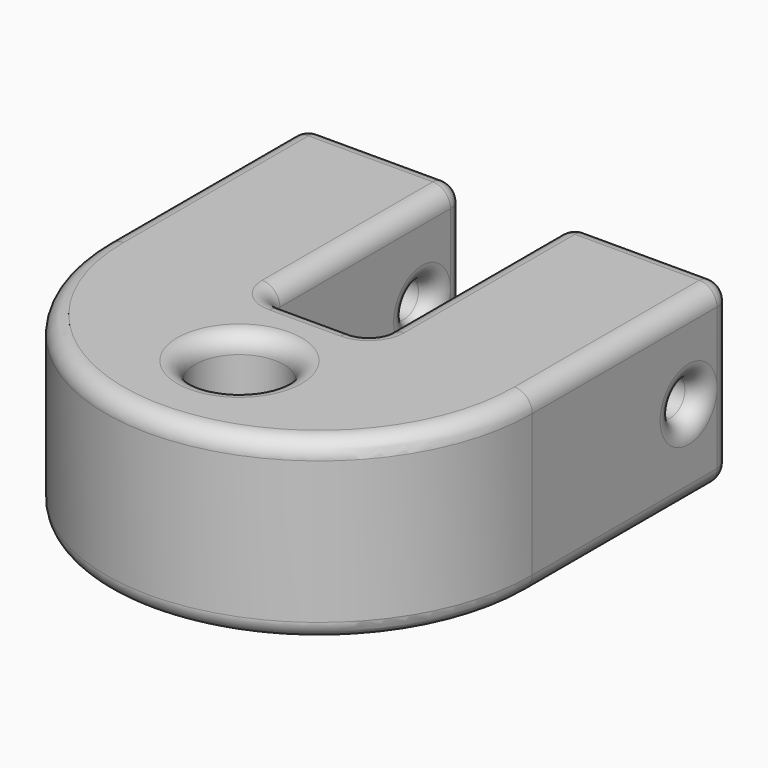
from build123d import *

# Parameters (mm, degrees)
F1_DEPTH = 50
F2_R     = 12.5
F3_DEPTH = 50.001
F4_R     = 5
F5_DEPTH = 120.001
F6_R     = 4.99999


# Not quite as in the source:
# - a fillet or chamfer is up to 0.001 mm smaller than in the source, because OpenCascade refuses the exact size


with BuildPart() as f1:
    # F0 (on Top) → F1 (new body)
    with BuildSketch(Plane.XY):
        with BuildLine():
            Line((-15, 70), (-60, 70))
            Line((-60, 70), (-60, 0))
            ThreePointArc((-60, 0), (0, -60), (60, 0))
            Line((60, 0), (60, 70))
            Line((60, 70), (15, 70))
            Line((15, 70), (15, 0))
            Line((15, 0), (-15, 0))
            Line((-15, 0), (-15, 70))
        make_face()
    extrude(amount=F1_DEPTH)

    # F2 (on face) → F3 (cut, through all)
    with BuildSketch(Plane.XY.offset(50)):
        with Locations((0, -28)):
            Circle(F2_R)
    extrude(amount=-F3_DEPTH, mode=Mode.SUBTRACT)

    # F4 (on face) → F5 (cut, through all)
    with BuildSketch(Plane.YZ.offset(60)):
        with Locations((55, 25)):
            Circle(F4_R)
    extrude(amount=-F5_DEPTH, mode=Mode.SUBTRACT)

    # F6 (radius 5 in the source; OpenCascade refuses exactly that, so slightly less here)
    f6_edges = [f1.edges().sort_by_distance(p)[0] for p in [
        (-12.5, -28, 50),
        (0, -60, 50),
        (0, 0, 50),
        (15, 0, 25),
        (-15, 0, 25),
        (0, 0, 0),
        (60, 70, 25),
        (15, 70, 25),
        (37.5, 70, 0),
        (37.5, 70, 50),
        (-15, 70, 25),
        (-60, 70, 25),
        (-37.5, 70, 0),
        (-37.5, 70, 50),
        (60, 35, 0),
        (0, -60, 0),
        (-60, 35, 0),
        (15, 35, 0),
        (-15, 35, 0),
        (-12.5, -28, 0),
        (-15, 50, 25),
        (-37.5, 60, 25),
        (-60, 50, 25),
        (60, 50, 25),
        (37.5, 60, 25),
        (15, 50, 25),
        (60, 35, 50),
        (-60, 35, 50),
        (15, 35, 50),
        (-15, 35, 50),
    ]]
    fillet(f6_edges, radius=F6_R)


solid = f1.part
